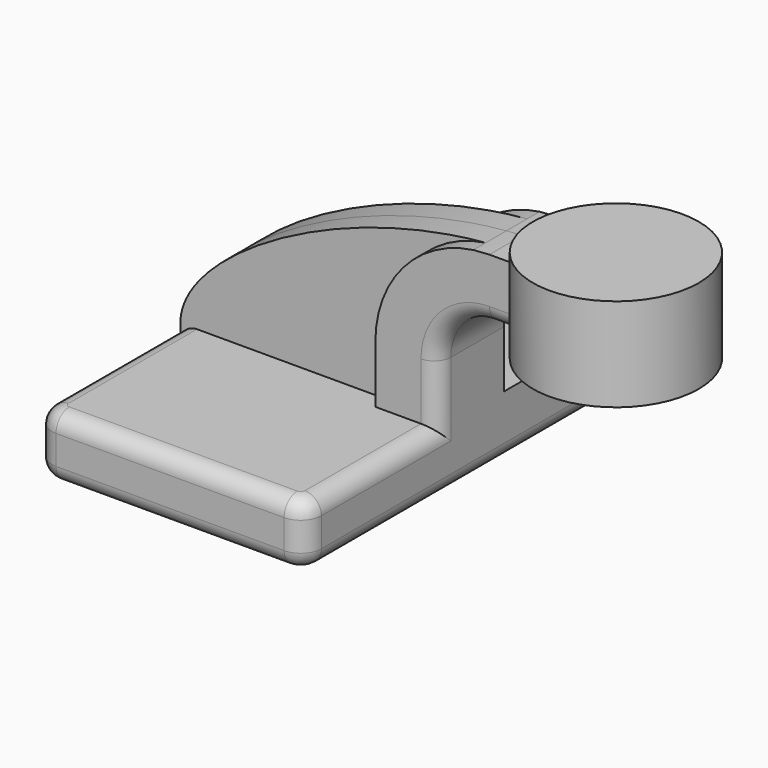
from build123d import *

# Parameters (mm, degrees)
F1_DEPTH     = 63.5
F0_W         = 25.4
F0_H         = 19.05
F2_DEPTH     = 12.7
F3_DEPTH     = 7.9375
F5_R         = 6.35
F6_T1_DEPTH  = 114.3
F6_T3_DEPTH  = 17.4752
F6_T5_DEPTH  = 49.2125
F6_T7_DEPTH  = 69.85
F6_T9_DEPTH  = 44.45
F6_T12_ANGLE = 90
F6_T14_ANGLE = 90
F6_T16_ANGLE = 90
F6_T18_ANGLE = 90
F6_T20_ANGLE = 90
F6_T22_ANGLE = 90
F6_T26_DEPTH = 19.2779547439
F6_S27_R     = 25.4
F6_T28_DEPTH = 12
F6_T30_ANGLE = 90
F6_T35_DEPTH = 57.15
F6_T39_DEPTH = 30.1752


# Not quite as in the source:
# - a fillet or chamfer that OpenCascade refuses, or shapes differently, is made with other operations: its cross-section is extruded or revolved along the edge and cut away or added


with BuildPart() as f1:
    # F0 (on Front) → F1 (new body, symmetric)
    with BuildSketch(Plane.XZ):
        Polygon((-41.275, 9.525), (-41.275, -9.525), (41.275, -9.525), (41.275, 9.525), (22.225, 9.525), align=None)
    extrude(amount=F1_DEPTH, both=True)

    # F0 (on Front) → F2 (join, symmetric)
    with BuildSketch(Plane.XZ):
        with BuildLine():
            Line((22.225, 9.525), (41.275, 9.525))
            Line((41.275, 9.525), (41.275, 27.0002))
            ThreePointArc((41.275, 27.0002), (45.9246798487, 38.2255201513), (57.15, 42.8752))
            Line((57.15, 42.8752), (60.325, 42.8752))
            Line((60.325, 42.8752), (60.325, 61.9252))
            Line((60.325, 61.9252), (57.15, 61.9252))
            add(Edge.make_bspline(
                [(52.2120910402, 61.5743620304), (53.8564284602, 61.7203088284), (55.5029986104, 61.8377030625), (57.15, 61.9252)],
                knots=[107.7945152041, 107.7945152041, 107.7945152041, 107.7945152041, 111.5045361635, 111.5045361635, 111.5045361635, 111.5045361635], degree=3))
            ThreePointArc((52.2120910402, 61.5743620304), (30.766178296, 49.8835908608), (22.225, 27.0002))
            Line((22.225, 27.0002), (22.225, 9.525))
        make_face()
        with Locations((73.025, 52.4002)):
            Rectangle(F0_W, F0_H)
    extrude(amount=F2_DEPTH, both=True)

    # F0 (on Front) → F3 (join, symmetric)
    with BuildSketch(Plane.XZ):
        with BuildLine():
            add(Edge.make_bspline(
                [(-41.275, 9.525), (-41.4553787608, 28.9895938663), (4.4359310246, 57.3338834698), (52.2120910402, 61.5743620304)],
                knots=[0, 0, 0, 0, 107.7945152041, 107.7945152041, 107.7945152041, 107.7945152041], degree=3))
            Line((-41.275, 9.525), (22.225, 9.525))
            Line((22.225, 9.525), (22.225, 27.0002))
            ThreePointArc((22.225, 27.0002), (30.766178296, 49.8835908608), (52.2120910402, 61.5743620304))
        make_face()
    extrude(amount=F3_DEPTH, both=True)

    # F0 (on Front) → F4 (revolve)
    with BuildSketch(Plane.XZ):
        Polygon((85.725, 66.675), (85.725, 61.9252), (85.725, 42.8752), (85.725, 38.1), (111.125, 38.1), (111.125, 66.675), align=None)
    revolve(axis=Axis((85.725, 0, 52.3875), (0, 0, -1)))

    # F5
    f5_edges = [f1.edges().sort_by_distance(p)[0] for p in [
        (41.275, -63.5, 0),
        (-41.275, -63.5, 0),
        (41.275, 63.5, 0),
        (-41.275, 63.5, 0),
    ]]
    fillet(f5_edges, radius=F5_R)

    # F6: fillet of radius 5.08 on 16 edges, made by hand

    # F6_s2 → F6_t1 (cut)
    with BuildSketch(Plane.XZ.offset(-57.15)):
        with BuildLine():
            ThreePointArc((36.195, -9.525), (39.7871024484, -8.0371024484), (41.275, -4.445))
            Line((41.275, -4.445), (41.275, -9.525))
            Line((41.275, -9.525), (36.195, -9.525))
        make_face()
        with BuildLine():
            ThreePointArc((-41.275, -4.445), (-39.7871024484, -8.0371024484), (-36.195, -9.525))
            Line((-36.195, -9.525), (-41.275, -9.525))
            Line((-41.275, -9.525), (-41.275, -4.445))
        make_face()
    extrude(amount=F6_T1_DEPTH, mode=Mode.SUBTRACT)

    # F6_s4 → F6_t3 (cut)
    with BuildSketch(Plane.XY.offset(9.525)):
        with BuildLine():
            ThreePointArc((41.275, -7.62), (39.7871024484, -11.2121024484), (36.195, -12.7))
            Line((36.195, -12.7), (41.275, -12.7))
            Line((41.275, -12.7), (41.275, -7.62))
        make_face()
    extrude(amount=F6_T3_DEPTH, mode=Mode.SUBTRACT)

    # F6_s6 → F6_t5 (cut)
    with BuildSketch(Plane.XZ.offset(7.9375)):
        with BuildLine():
            ThreePointArc((-41.275, 4.445), (-39.7871024484, 8.0371024484), (-36.195, 9.525))
            Line((-36.195, 9.525), (-41.275, 9.525))
            Line((-41.275, 9.525), (-41.275, 4.445))
        make_face()
    extrude(amount=F6_T5_DEPTH, mode=Mode.SUBTRACT)

    # F6_s8 → F6_t7 (cut)
    with BuildSketch(Plane.YZ.offset(-34.925)):
        with BuildLine():
            ThreePointArc((58.42, -9.525), (62.0121024484, -8.0371024484), (63.5, -4.445))
            Line((63.5, -4.445), (63.5, -9.525))
            Line((63.5, -9.525), (58.42, -9.525))
        make_face()
        with BuildLine():
            ThreePointArc((-58.42, -9.525), (-62.0121024484, -8.0371024484), (-63.5, -4.445))
            Line((-63.5, -4.445), (-63.5, -9.525))
            Line((-63.5, -9.525), (-58.42, -9.525))
        make_face()
        with BuildLine():
            ThreePointArc((-58.42, 9.525), (-62.0121024484, 8.0371024484), (-63.5, 4.445))
            Line((-63.5, 4.445), (-63.5, 9.525))
            Line((-63.5, 9.525), (-58.42, 9.525))
        make_face()
    extrude(amount=F6_T7_DEPTH, mode=Mode.SUBTRACT)

    # F6_s10 → F6_t9 (cut)
    with BuildSketch(Plane.XZ.offset(12.7)):
        with BuildLine():
            ThreePointArc((36.195, 9.525), (39.7871024484, 8.0371024484), (41.275, 4.445))
            Line((41.275, 4.445), (41.275, 9.525))
            Line((41.275, 9.525), (36.195, 9.525))
        make_face()
    extrude(amount=F6_T9_DEPTH, mode=Mode.SUBTRACT)

    # F6_s11 → F6_t12 (revolve, cut)
    with BuildSketch(Plane.YZ.offset(34.925)):
        with BuildLine():
            ThreePointArc((-58.42, 9.525), (-62.0121024484, 8.0371024484), (-63.5, 4.445))
            Line((-63.5, 4.445), (-63.5, 9.525))
            Line((-63.5, 9.525), (-58.42, 9.525))
        make_face()
    revolve(axis=Axis((34.925, -57.15, 9.525), (0, 0, 1)), revolution_arc=F6_T12_ANGLE, mode=Mode.SUBTRACT)

    # F6_s13 → F6_t14 (revolve, cut)
    with BuildSketch(Plane.XZ.offset(-57.15)):
        with BuildLine():
            ThreePointArc((-36.195, -9.525), (-39.7871024484, -8.0371024484), (-41.275, -4.445))
            Line((-41.275, -4.445), (-41.275, -9.525))
            Line((-41.275, -9.525), (-36.195, -9.525))
        make_face()
    revolve(axis=Axis((-34.925, 57.15, -9.525), (0, 0, -1)), revolution_arc=F6_T14_ANGLE, mode=Mode.SUBTRACT)

    # F6_s15 → F6_t16 (revolve, cut)
    with BuildSketch(Plane.XZ.offset(57.15)):
        with BuildLine():
            ThreePointArc((-36.195, -9.525), (-39.7871024484, -8.0371024484), (-41.275, -4.445))
            Line((-41.275, -4.445), (-41.275, -9.525))
            Line((-41.275, -9.525), (-36.195, -9.525))
        make_face()
    revolve(axis=Axis((-34.925, -57.15, -9.525), (0, 0, 1)), revolution_arc=F6_T16_ANGLE, mode=Mode.SUBTRACT)

    # F6_s17 → F6_t18 (revolve, cut)
    with BuildSketch(Plane.YZ.offset(34.925)):
        with BuildLine():
            ThreePointArc((58.42, -9.525), (62.0121024484, -8.0371024484), (63.5, -4.445))
            Line((63.5, -4.445), (63.5, -9.525))
            Line((63.5, -9.525), (58.42, -9.525))
        make_face()
    revolve(axis=Axis((34.925, 57.15, -9.525), (0, 0, -1)), revolution_arc=F6_T18_ANGLE, mode=Mode.SUBTRACT)

    # F6_s19 → F6_t20 (revolve, cut)
    with BuildSketch(Plane.YZ.offset(34.925)):
        with BuildLine():
            ThreePointArc((-58.42, -9.525), (-62.0121024484, -8.0371024484), (-63.5, -4.445))
            Line((-63.5, -4.445), (-63.5, -9.525))
            Line((-63.5, -9.525), (-58.42, -9.525))
        make_face()
    revolve(axis=Axis((34.925, -57.15, -9.525), (0, 0, 1)), revolution_arc=F6_T20_ANGLE, mode=Mode.SUBTRACT)

    # F6_s21 → F6_t22 (revolve, cut)
    with BuildSketch(Plane.XZ.offset(57.15)):
        with BuildLine():
            ThreePointArc((-41.275, 4.445), (-39.7871024484, 8.0371024484), (-36.195, 9.525))
            Line((-36.195, 9.525), (-41.275, 9.525))
            Line((-41.275, 9.525), (-41.275, 4.445))
        make_face()
    revolve(axis=Axis((-34.925, -57.15, 9.525), (0, 0, 1)), revolution_arc=F6_T22_ANGLE, mode=Mode.SUBTRACT)


with BuildPart() as f6_tool24:
    # F6_s25 → F6_t26 (new body)
    with BuildSketch(Plane.YZ.offset(57.15)):
        with BuildLine():
            ThreePointArc((-12.7, 47.9552), (-11.2121024484, 44.3630975516), (-7.62, 42.8752))
            Line((-7.62, 42.8752), (-12.7, 42.8752))
            Line((-12.7, 42.8752), (-12.7, 47.9552))
        make_face()
    extrude(amount=F6_T26_DEPTH)

    # F6_s27 → F6_t28 (cut, symmetric)
    with BuildSketch(Plane.XY.offset(45.4)):
        with Locations((85.725, 0)):
            Circle(F6_S27_R)
    extrude(amount=F6_T28_DEPTH, both=True, mode=Mode.SUBTRACT)


with BuildPart() as f1_1:
    add(f1.part)

    # F6_t23: cut F6_tool24
    add(f6_tool24.part, mode=Mode.SUBTRACT)

    # F6_s29 → F6_t30 (revolve, cut)
    with BuildSketch(Plane.XY.offset(27.0002)):
        with BuildLine():
            ThreePointArc((36.195, -12.7), (39.7871024484, -11.2121024484), (41.275, -7.62))
            Line((41.275, -7.62), (41.275, -12.7))
            Line((41.275, -12.7), (36.195, -12.7))
        make_face()
    revolve(axis=Axis((57.15, -12.7, 27.0002), (0, 1, 0)), revolution_arc=F6_T30_ANGLE, mode=Mode.SUBTRACT)


with BuildPart() as f6_tool33:
    # F6_s34 → F6_t35 (new body)
    with BuildSketch(Plane.XZ.offset(57.15)):
        with BuildLine():
            ThreePointArc((36.195, 9.525), (39.7871024484, 8.0371024484), (41.275, 4.445))
            Line((41.275, 4.445), (41.275, 9.525))
            Line((41.275, 9.525), (36.195, 9.525))
        make_face()
    extrude(amount=-F6_T35_DEPTH)

    split(bisect_by=Plane.XZ.offset(12.7), keep=Keep.BOTTOM)


with BuildPart() as f6_tool37:
    # F6_s38 → F6_t39 (new body)
    with BuildSketch(Plane.XY.offset(-3.175)):
        with BuildLine():
            ThreePointArc((41.275, -7.62), (39.7871024484, -11.2121024484), (36.195, -12.7))
            Line((36.195, -12.7), (41.275, -12.7))
            Line((41.275, -12.7), (41.275, -7.62))
        make_face()
    extrude(amount=F6_T39_DEPTH)

    split(bisect_by=Plane.XY.offset(9.525), keep=Keep.BOTTOM)


with BuildPart() as f6_tool33_1:
    add(f6_tool33.part)

    # F6_t41: intersect F6_tool37
    add(f6_tool37.part, mode=Mode.INTERSECT)


with BuildPart() as f1_2:
    add(f1_1.part)

    # F6_t31: cut F6_tool33
    add(f6_tool33_1.part, mode=Mode.SUBTRACT)


solid = f1_2.part
